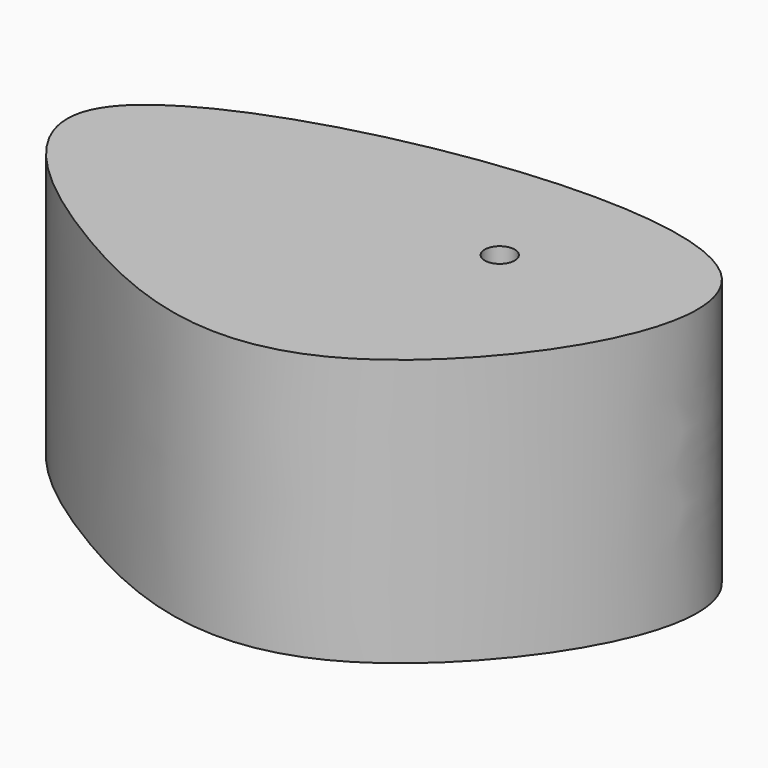
from build123d import *

# Parameters (mm, degrees)
F1_DEPTH = 56.61061
F4_D     = 6.35


# Not quite as in the source:
# - the program builds the solid bodies; features that only make, move or delete a surface that nothing else refers to are left out


with BuildPart() as f1:
    # F0 (on Top) → F1 (new body)
    with BuildSketch(Plane.XY):
        with BuildLine():
            add(Edge.make_bspline(
                [(-76.1927515268, -11.1532108858), (-94.4367577585, -0.4668757066), (-143.1214573776, 38.7984332094), (56.6380279203, 75.270590056), (-15.4747114675, -35.8843276344), (-55.7508781473, -23.1269357273), (-76.1927515268, -11.1532108858)],
                knots=[0, 0, 0, 0, 0.2050451004, 0.5264276013, 0.7702529846, 1, 1, 1, 1], degree=3))
        make_face()
    extrude(amount=F1_DEPTH)

    # F4 (through all)
    with Locations(Plane.XY.offset(56.61061)):
        with Locations((-20.2039089054, 27.292644605)):
            Hole(F4_D / 2)


solid = f1.part
